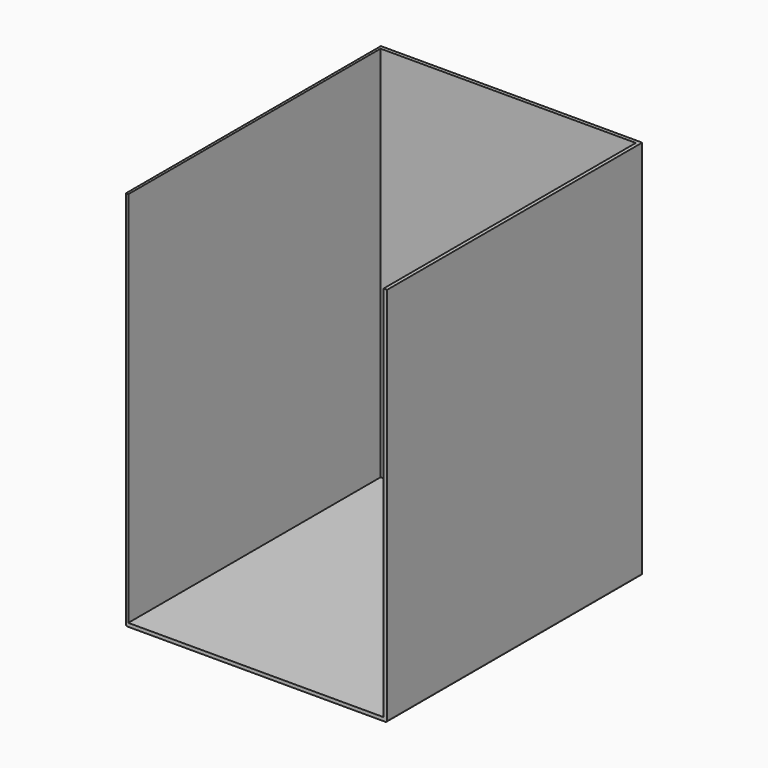
from build123d import *

# Parameters (mm, degrees)
F1_DEPTH = 426
F2_W     = 295
F2_H     = 360
F3_DEPTH = 4
F4_R     = 2


# Not quite as in the source:
# - a feature names something its author has since deleted; it is built from what else it names


with BuildPart() as f1:
    # F0 (on Top) → F1 (new body)
    with BuildSketch(Plane.XY):
        Polygon((-4, -360), (0, -360), (0, 0), (-295, 0), (-295, -360), (-292.1838745495, -360), (-292.1838745495, -4), (-4, -4), align=None)
    extrude(amount=F1_DEPTH)

    # F2 (on Top) → F3 (join)
    with BuildSketch(Plane.XY):
        with Locations((-147.5, -180)):
            Rectangle(F2_W, F2_H)
    extrude(amount=-F3_DEPTH)

    # F4
    f4_edges = [f1.edges().sort_by_distance(p)[0] for p in [
        (0, -180, -4),
        (-295, -180, -4),
        (-147.5, 0, -4),
    ]]
    fillet(f4_edges, radius=F4_R)


solid = f1.part
